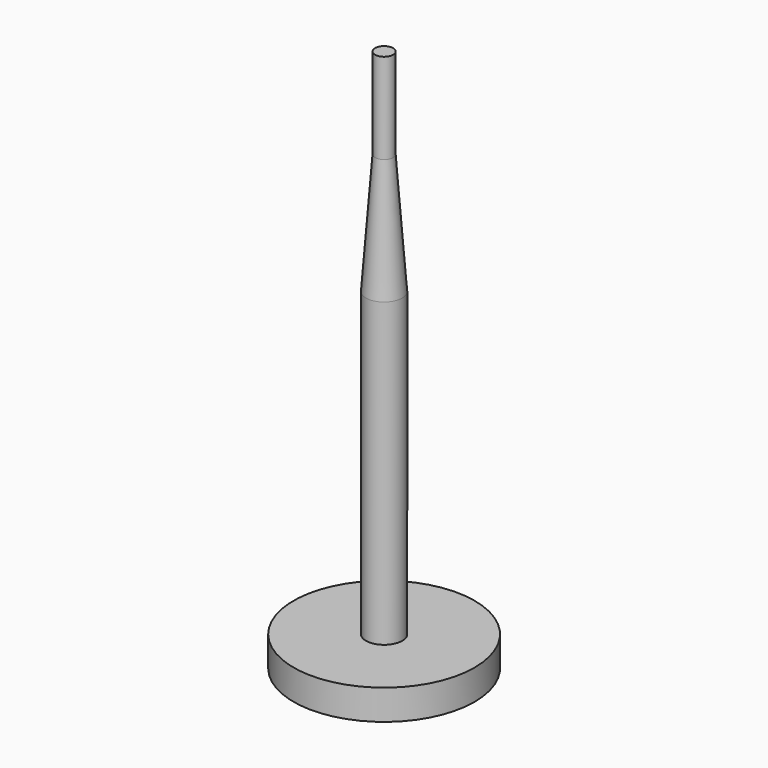
from build123d import *

# Parameters (mm, degrees)
F0_R     = 38.1
F1_DEPTH = 12.7
F2_R     = 7.62
F3_DEPTH = 127
F6_DEPTH = 38.1


# Not quite as in the source:
# - a feature names something its author has since deleted; it is built from what else it names


with BuildPart() as f1:
    # F0 (on Top) → F1 (new body)
    with BuildSketch(Plane.XY):
        Circle(F0_R)
    extrude(amount=F1_DEPTH)

    # F2 (on face) → F3 (join)
    with BuildSketch(Plane.XY.offset(12.7)):
        Circle(F2_R)
    extrude(amount=F3_DEPTH)

    # F4 (on Right) → F5 (revolve)
    with BuildSketch(Plane.YZ):
        Polygon((0, 190.5), (0, 139.7), (7.62, 139.7), (3.81, 190.5), align=None)
    revolve(axis=Axis((0, 0, 165.1), (0, 0, 1)))

    # F6 (add): a face of the model
    f6_faces = [f1.faces().sort_by_distance(p)[0] for p in [
        (0, 0, 190.5),
    ]]
    extrude(f6_faces, amount=F6_DEPTH)


solid = f1.part
